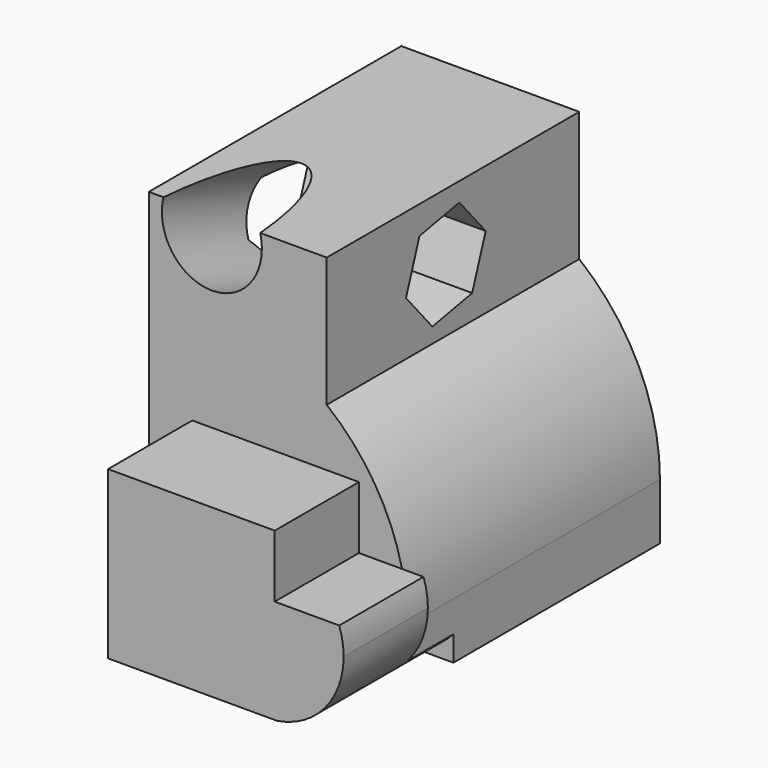
from build123d import *

# Parameters (mm, degrees)
F0_W          = 62.0737820864
F0_H          = 75.7545232773
F1_DEPTH      = 53.8003519177
F2_W          = 42.7050869912
F2_H          = 75.7545232773
F3_DEPTH      = 31.1090257019
F5_DEPTH      = 50.4763200879
F6_R          = 11.9924338382
F7_DEPTH      = 57.1455173194
F7_DEPTH_BACK = 70.5328881741
F8_W          = 23.3642431419
F8_H          = 25
F9_DEPTH      = 25.2702012658
F11_DEPTH     = 39.0601754189
F12_T1_DEPTH  = 176.500859237


# Not quite as in the source:
# - a fillet or chamfer that OpenCascade refuses, or shapes differently, is made with other operations: its cross-section is extruded or revolved along the edge and cut away or added


with BuildPart() as f1:
    # F0 (on Top) → F1 (new body)
    with BuildSketch(Plane.XY):
        with Locations((3.4712180495, 2.1439939737)):
            Rectangle(F0_W, F0_H)
    extrude(amount=F1_DEPTH)

    # F2 (on face) → F3 (join)
    with BuildSketch(Plane.XY.offset(53.8003519177)):
        with Locations((-6.2131294981, 2.1439939737)):
            Rectangle(F2_W, F2_H)
    extrude(amount=F3_DEPTH)

    # F4 (on face) → F5 (cut)
    with BuildSketch(Plane.YZ.offset(15.1394139975)):
        Polygon((7.902597892, 59.6732337929), (11.9554921985, 71.1383074522), (4.0528943065, 80.3807537101), (-7.902597892, 78.1581263088), (-11.9554921985, 66.6930526495), (-4.0528943065, 57.4506063916), align=None)
    extrude(amount=-F5_DEPTH, mode=Mode.SUBTRACT)

    # F6 (on face) → F7 (cut, two sides)
    with BuildSketch(Plane(origin=(0, -11.726481381, 4.1453017256), x_dir=(1, 0, 0), z_dir=(0, -0.9428250988, 0.3332879132))) as f7_sk:
        with Locations((-12.427136302, 65.1199892163)):
            Circle(F6_R)
    extrude(amount=-F7_DEPTH, mode=Mode.SUBTRACT)
    extrude(f7_sk.sketch, amount=F7_DEPTH_BACK, mode=Mode.SUBTRACT)

    # F8 (on face) → F9 (join)
    with BuildSketch(Plane.XZ.offset(35.7332676649)):
        with Locations((46.1902306637, 12.5)):
            Rectangle(F8_W, F8_H)
        Polygon((-17.1276477654, 40), (-17.1276477654, 0), (34.5081090927, 0), (34.5081090927, 25), (22.8723522346, 25), (22.8723522346, 40), align=None)
    extrude(amount=F9_DEPTH)

    # F10 (on face) → F11 (cut)
    with BuildSketch(Plane.XZ.offset(61.0034689307)):
        with BuildLine():
            ThreePointArc((38.360852409, 25), (39.1514020631, 21.9206371156), (39.417401399, 18.7525637448))
            ThreePointArc((39.417401399, 18.7525637448), (34.8909952827, 6.443784061), (23.4685587384, 0))
            Line((23.4685587384, 0), (57.8723522346, 0))
            Line((57.8723522346, 0), (57.8723522346, 25))
            Line((57.8723522346, 25), (38.360852409, 25))
        make_face()
    extrude(amount=-F11_DEPTH, mode=Mode.SUBTRACT)

    # F12: fillet of radius 51.606941339 on 1 edges, made by hand

    # F12_s2 → F12_t1 (cut)
    with BuildSketch(Plane.XZ.offset(-140.7675915721)):
        with BuildLine():
            ThreePointArc((34.5081090927, 13.5018175338), (29.4145726879, 35.8575674831), (15.1394139975, 53.8003519177))
            Line((15.1394139975, 53.8003519177), (34.5081090927, 53.8003519177))
            Line((34.5081090927, 53.8003519177), (34.5081090927, 13.5018175338))
        make_face()
    extrude(amount=F12_T1_DEPTH, mode=Mode.SUBTRACT)


solid = f1.part
